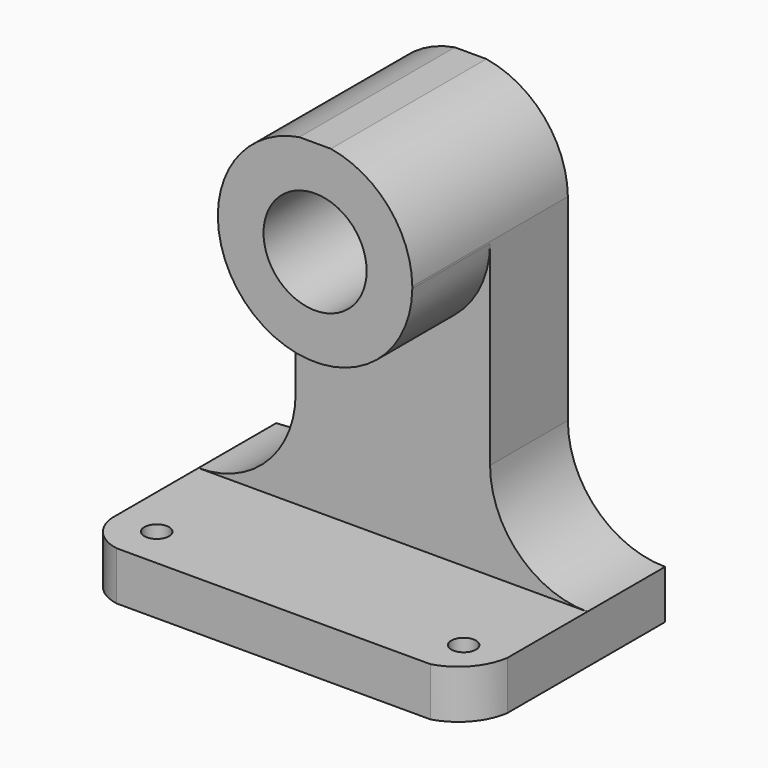
from build123d import *

# Parameters (mm, degrees)
F0_W      = 50.8
F0_H      = 57.15
F1_DEPTH  = 31.75
F3_DEPTH  = 50.8
F4_W      = 12.7
F4_H      = 25.4
F5_DEPTH  = 25.4
F6_W      = 12.7
F6_H      = 12.7
F7_DEPTH  = 25.4
F9_DEPTH  = 25.4
F11_DEPTH = 25.4
F13_DEPTH = 12.7
F14_R     = 6.7335002537
F15_DEPTH = 25.4
F17_DEPTH = 25.4
F18_R     = 1.6140947443
F18_R_2   = 1.6110130755
F19_DEPTH = 25.4


with BuildPart() as f1:
    # F0 (on Front) → F1 (new body)
    with BuildSketch(Plane.XZ):
        with Locations((-43.8855561577, 28.575)):
            Rectangle(F0_W, F0_H)
    extrude(amount=F1_DEPTH)

    # F2 (on face) → F3 (cut)
    with BuildSketch(Plane(origin=(-69.2855561577, 0, 0), x_dir=(0, -1, 0), z_dir=(-1, 0, 0))):
        Polygon((12.7, 6.35), (31.75, 6.35), (31.75, 57.15), (25.4, 57.15), (25.4, 31.75), (12.7, 31.75), align=None)
    extrude(amount=-F3_DEPTH, mode=Mode.SUBTRACT)

    # F4 (on face) → F5 (cut)
    with BuildSketch(Plane.XZ.offset(25.4)):
        with Locations((-24.8355561577, 44.45)):
            Rectangle(F4_W, F4_H)
        with Locations((-62.9355561577, 44.45)):
            Rectangle(F4_W, F4_H)
    extrude(amount=-F5_DEPTH, mode=Mode.SUBTRACT)

    # F6 (on face) → F7 (cut)
    with BuildSketch(Plane.XZ.offset(12.7)):
        with Locations((-62.9355561577, 25.4)):
            Rectangle(F6_W, F6_H)
        with Locations((-24.8355561577, 25.4)):
            Rectangle(F6_W, F6_H)
    extrude(amount=-F7_DEPTH, mode=Mode.SUBTRACT)

    # F8 (on face) → F9 (cut)
    with BuildSketch(Plane.XZ.offset(12.7)):
        with BuildLine():
            Line((-69.2855561577, 19.05), (-69.2855561577, 6.35))
            ThreePointArc((-69.2855561577, 6.35), (-60.3053000366, 10.0697438789), (-56.5855561577, 19.05))
            Line((-56.5855561577, 19.05), (-69.2855561577, 19.05))
        make_face()
        with BuildLine():
            ThreePointArc((-31.1855561577, 19.05), (-27.4658122788, 10.0697438789), (-18.4855561577, 6.35))
            Line((-18.4855561577, 6.35), (-18.4855561577, 19.05))
            Line((-18.4855561577, 19.05), (-31.1855561577, 19.05))
        make_face()
    extrude(amount=-F9_DEPTH, mode=Mode.SUBTRACT)

    # F10 (on face) → F11 (cut)
    with BuildSketch(Plane.XZ.offset(25.4)):
        with BuildLine():
            Line((-56.5855561577, 57.15), (-56.5855561577, 44.7837235148))
            ThreePointArc((-56.5855561577, 44.7837235148), (-53.5129172667, 52.9012905804), (-45.9442665885, 57.15))
            Line((-45.9442665885, 57.15), (-56.5855561577, 57.15))
        make_face()
        with BuildLine():
            ThreePointArc((-41.8268457269, 57.15), (-34.2581950488, 52.9012905804), (-31.1855561577, 44.7837235148))
            Line((-31.1855561577, 44.7837235148), (-31.1855561577, 57.15))
            Line((-31.1855561577, 57.15), (-41.8268457269, 57.15))
        make_face()
    extrude(amount=-F11_DEPTH, mode=Mode.SUBTRACT)

    # F12 (on face) → F13 (cut)
    with BuildSketch(Plane.XZ.offset(25.4)):
        with BuildLine():
            ThreePointArc((-31.1855561577, 44.5365372296), (-43.8855561577, 31.9595289981), (-56.5855561577, 44.5365372296))
            Line((-56.5855561577, 44.5365372296), (-56.5855561577, 31.75))
            Line((-56.5855561577, 31.75), (-31.1855561577, 31.75))
            Line((-31.1855561577, 31.75), (-31.1855561577, 44.5365372296))
        make_face()
    extrude(amount=-F13_DEPTH, mode=Mode.SUBTRACT)

    # F14 (on face) → F15 (cut)
    with BuildSketch(Plane.XZ.offset(25.4)):
        with Locations((-43.8855561577, 44.6168617574)):
            Circle(F14_R)
    extrude(amount=-F15_DEPTH, mode=Mode.SUBTRACT)

    # F16 (on face) → F17 (cut)
    with BuildSketch(Plane.XY.offset(6.35)):
        with BuildLine():
            ThreePointArc((-64.719619815, -31.75), (-67.8220929264, -30.0962429481), (-69.2855561577, -26.8995998395))
            Line((-69.2855561577, -26.8995998395), (-69.2855561577, -31.75))
            Line((-69.2855561577, -31.75), (-64.719619815, -31.75))
        make_face()
        with BuildLine():
            Line((-18.4855561577, -31.75), (-18.4855561577, -25.7653463632))
            ThreePointArc((-18.4855561577, -25.7653463632), (-20.2347846396, -29.5237639054), (-23.7318370491, -31.75))
            Line((-23.7318370491, -31.75), (-18.4855561577, -31.75))
        make_face()
    extrude(amount=-F17_DEPTH, mode=Mode.SUBTRACT)

    # F18 (on face) → F19 (cut)
    with BuildSketch(Plane.XY.offset(6.35)):
        with Locations((-63.8238352858, -26.3324731014)):
            Circle(F18_R)
        with Locations((-23.7318370491, -26.3324731014)):
            Circle(F18_R_2)
    extrude(amount=-F19_DEPTH, mode=Mode.SUBTRACT)


solid = f1.part
